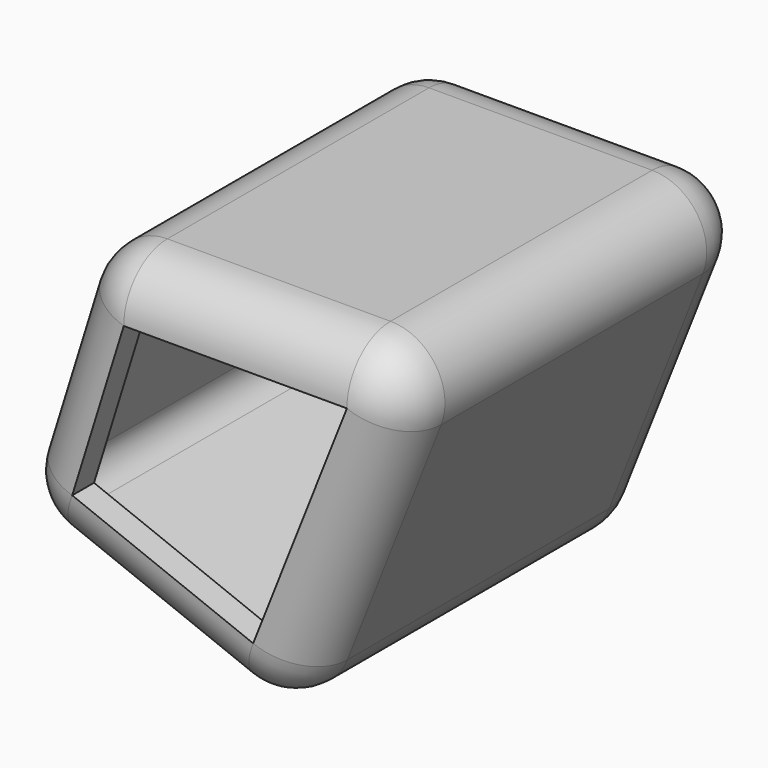
from build123d import *

# Parameters (mm, degrees)
F1_DEPTH = 50.8
F2_R     = 12.7
F3_T     = -6.35


# Not quite as in the source:
# - a shell that OpenCascade refuses in one call is made with other operations: the cavity is built on its own and cut out


with BuildPart() as f1:
    # F0 (on Front) → F1 (new body, symmetric)
    with BuildSketch(Plane.XZ):
        Polygon((36.0003995515, 21.6075032949), (-44.0155640244, 21.6075032949), (-62.2989119761, -37.2344391203), (2.6374720037, -62.877625227), align=None)
    extrude(amount=F1_DEPTH, both=True)

    # F2
    f2_edges = [f1.edges().sort_by_distance(p)[0] for p in [
        (36.0004, 0, 21.607503),
        (-4.007582, 50.8, 21.607503),
        (-44.015564, 0, 21.607503),
        (-4.007582, -50.8, 21.607503),
        (19.318936, -50.8, -20.635061),
        (-53.157238, -50.8, -7.813468),
        (-29.83072, -50.8, -50.056032),
        (19.318936, 50.8, -20.635061),
        (2.637472, 0, -62.877625),
        (-53.157238, 50.8, -7.813468),
        (-29.83072, 50.8, -50.056032),
        (-62.298912, 0, -37.234439),
    ]]
    fillet(f2_edges, radius=F2_R)

    # F3: a shell. OpenCascade refuses it in one call, so the cavity is built on its own and cut out:
    # the body offset inwards by the wall thickness, plus a prism from it out through each open face.
    f3_core = offset(f1.part, amount=F3_T, mode=Mode.PRIVATE)
    f3_exits = [f3_core.faces().sort_by_distance(p)[0] for p in [
        (-15.577686, -44.45, -14.539718),
    ]]
    add(f3_core, mode=Mode.SUBTRACT)
    extrude(f3_exits, amount=-F3_T, mode=Mode.SUBTRACT)


solid = f1.part
